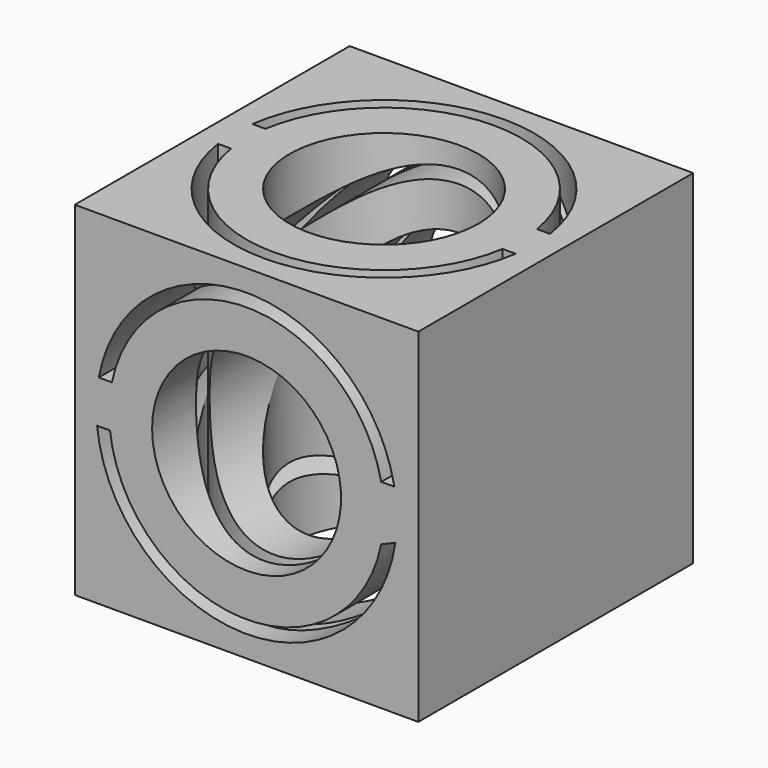
from build123d import *

# Parameters (mm, degrees)
F0_R     = 11
F1_DEPTH = 40
F2_R     = 11
F3_DEPTH = 40


# Not quite as in the source:
# - a feature of the source that left no trace in its solid (it failed there, or was rolled back) is left out


with BuildPart() as f1:
    # F0 (on Top) → F1 (new body)
    with BuildSketch(Plane.XY):
        Polygon((-20, -20), (0, -20), (20, -20), (20, 0), (20, 20), (0, 20), (-20, 20), (-20, 0), align=None)
        with BuildLine():
            Line((-17.3205080757, -2.5), (-15.8034806293, -2.5))
            ThreePointArc((-15.8034806293, -2.5), (0, -16), (15.8034806293, -2.5))
            Line((15.8034806293, -2.5), (17.3205080757, -2.5))
            ThreePointArc((17.3205080757, -2.5), (0, -17.5), (-17.3205080757, -2.5))
        make_face(mode=Mode.SUBTRACT)
        Circle(F0_R, mode=Mode.SUBTRACT)
        with BuildLine():
            Line((-15.8034806293, 2.5), (-17.3205080757, 2.5))
            ThreePointArc((-17.3205080757, 2.5), (0, 17.5), (17.3205080757, 2.5))
            Line((17.3205080757, 2.5), (15.8034806293, 2.5))
            ThreePointArc((15.8034806293, 2.5), (0, 16), (-15.8034806293, 2.5))
        make_face(mode=Mode.SUBTRACT)
    extrude(amount=F1_DEPTH)

    # F2 (on face) → F3 (cut)
    with BuildSketch(Plane(origin=(0, 20, 0), x_dir=(-1, 0, 0), z_dir=(0, 1, 0))):
        with Locations((0, 20)):
            Circle(F2_R)
        with BuildLine():
            ThreePointArc((15.8984275952, 18.2), (0.7087220706, 4.0157041748), (-15.6767343538, 16.8))
            Line((-15.6767343538, 16.8), (-17.3205080757, 17.5))
            ThreePointArc((-17.3205080757, 17.5), (0.3526728097, 2.5035540212), (17.4071824257, 18.2))
            Line((17.4071824257, 18.2), (15.8984275952, 18.2))
        make_face()
        with BuildLine():
            ThreePointArc((17.2049411507, 23.2), (0, 37.5), (-17.2049411507, 23.2))
            Line((-17.2049411507, 23.2), (-15.6767343538, 23.2))
            ThreePointArc((-15.6767343538, 23.2), (0, 36), (15.6767343538, 23.2))
            Line((15.6767343538, 23.2), (17.2049411507, 23.2))
        make_face()
    extrude(amount=-F3_DEPTH, mode=Mode.SUBTRACT)


solid = f1.part
